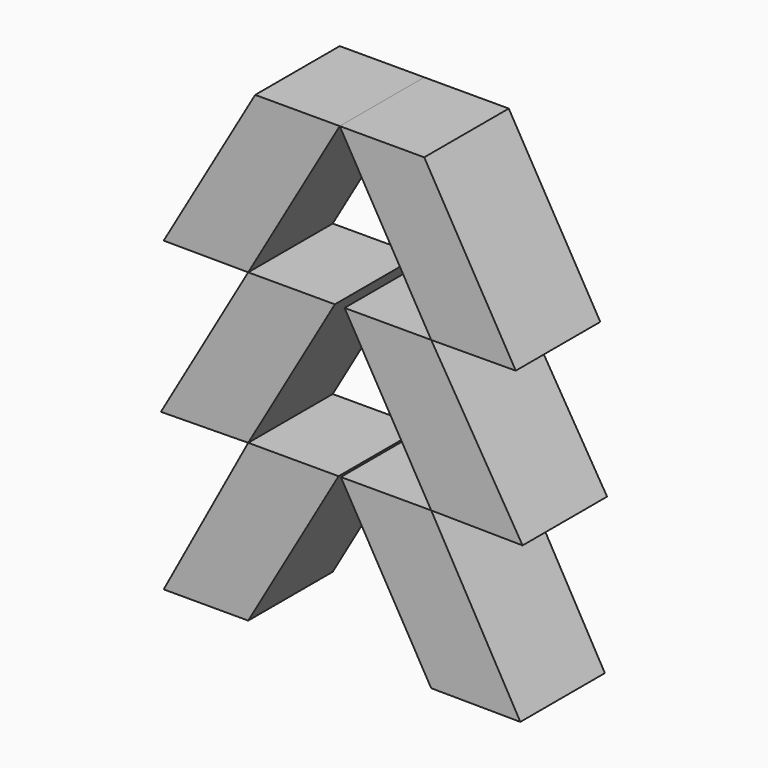
from build123d import *

# Parameters (mm, degrees)
F1_DEPTH = 12.7


# Not quite as in the source:
# - a length typed as a fraction of an inch, garbled in the dataset ("3 / 203.2 mm" for 3/8 in), is restored


with BuildPart() as f1:
    # F0 (on Front) → F1 (new body)
    with BuildSketch(Plane.XZ):
        Polygon((-10.9985226281, -6.35), (0, 12.7), (-10.16, 12.7), (-21.1585226281, -6.2996095111), align=None)
    extrude(amount=F1_DEPTH)


with BuildPart() as f1b:
    # F0 (on Front) → F1, piece 2 (new body)
    with BuildSketch(Plane.XZ):
        Polygon((10.16, 12.7), (0, 12.7), (10.9985226281, -6.35), (21.1585226281, -6.2996095111), align=None)
    extrude(amount=F1_DEPTH)


with BuildPart() as f1c:
    # F0 (on Front) → F1, piece 3 (new body)
    with BuildSketch(Plane.XZ):
        Polygon((-0.5832433259, -6.35), (-10.9985226281, -6.35), (-21.4922550901, -24.5256777853), (-10.9985226281, -24.3897929265), align=None)
    extrude(amount=F1_DEPTH)


with BuildPart() as f1d:
    # F0 (on Front) → F1, piece 4 (new body)
    with BuildSketch(Plane.XZ):
        Polygon((21.9792984426, -24.5256777853), (10.9985226281, -6.35), (0.5832433259, -6.35), (10.9985226281, -24.3897929265), align=None)
    extrude(amount=F1_DEPTH)


with BuildPart() as f1e:
    # F0 (on Front) → F1, piece 5 (new body)
    with BuildSketch(Plane.XZ):
        Polygon((-0.1352517672, -24.3897929265), (-10.9985226281, -24.3897929265), (-21.1585226281, -43.2055299938), (-10.9985226281, -43.2055299938), align=None)
    extrude(amount=F1_DEPTH)


with BuildPart() as f1f:
    # F0 (on Front) → F1, piece 6 (new body)
    with BuildSketch(Plane.XZ):
        Polygon((21.7112582177, -43.2884916663), (10.9985226281, -24.3897929265), (0.1352517672, -24.3897929265), (10.9985226281, -43.2055299938), align=None)
    extrude(amount=F1_DEPTH)


solid = Compound([f1.part, f1b.part, f1c.part, f1d.part, f1e.part, f1f.part])
